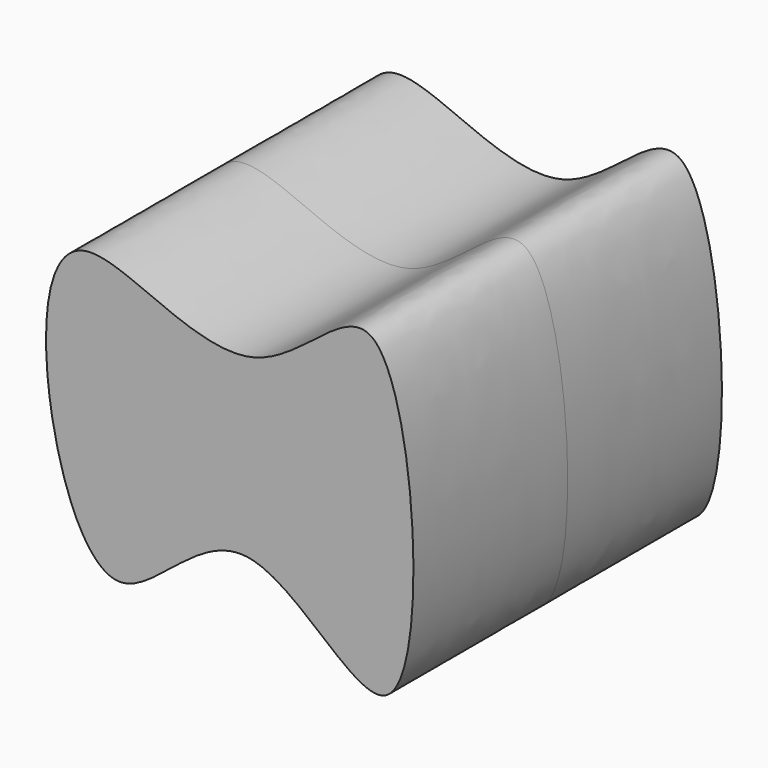
from build123d import *

# Parameters (mm, degrees)
F1_DEPTH = 38.1


# Not quite as in the source:
# - the program builds the solid bodies; features that only make, move or delete a surface that nothing else refers to are left out


with BuildPart() as f1:
    # F0 (on Front) → F1 (new body, symmetric)
    with BuildSketch(Plane.XZ):
        with BuildLine():
            add(Edge.make_bspline(
                [(-30.508486554, 11.5154581144), (-31.6019733126, 23.8463236007), (-27.304289442, 46.6380760277), (10.6742573925, 14.8568561254), (40.6187456041, 63.5607828107), (47.0797908255, -51.3764017647), (8.0015721275, 8.3361382392), (-18.7338734511, -35.0859230495), (-29.225118154, -2.9566358411), (-30.508486554, 11.5154581144)],
                knots=[0, 0, 0, 0, 0.123426007, 0.2667582283, 0.3933298593, 0.5860028181, 0.7251133668, 0.8551413304, 1, 1, 1, 1], degree=3))
        make_face()
    extrude(amount=F1_DEPTH, both=True)


solid = f1.part
